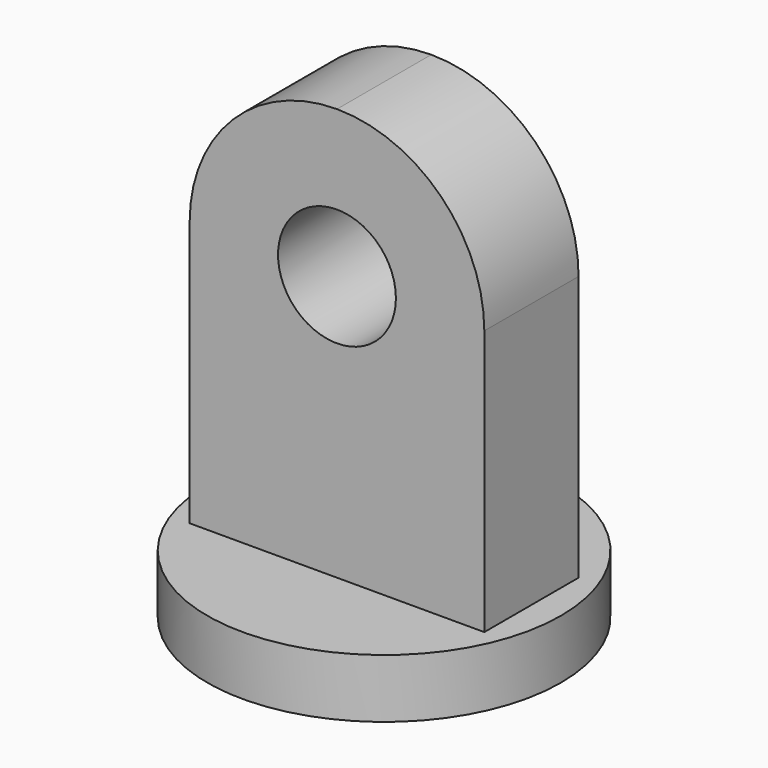
from build123d import *

# Parameters (mm, degrees)
F0_R     = 3
F1_DEPTH = 1
F2_W     = 5
F2_H     = 2
F3_DEPTH = 7
F4_R     = 2.49999
F5_R     = 1
F6_DEPTH = 4


# Not quite as in the source:
# - a fillet or chamfer is up to 0.001 mm smaller than in the source, because OpenCascade refuses the exact size


with BuildPart() as f1:
    # F0 (on Top) → F1 (new body)
    with BuildSketch(Plane.XY):
        Circle(F0_R)
    extrude(amount=F1_DEPTH)

    # F2 (on face) → F3 (join)
    with BuildSketch(Plane.XY.offset(1)):
        Rectangle(F2_W, F2_H)
    extrude(amount=F3_DEPTH)

    # F4 (radius 2.5 in the source; OpenCascade refuses exactly that, so slightly less here)
    f4_edges = [f1.edges().sort_by_distance(p)[0] for p in [
        (-2.5, 0, 8),
        (2.5, 0, 8),
    ]]
    fillet(f4_edges, radius=F4_R)

    # F5 (on face) → F6 (cut)
    with BuildSketch(Plane.XZ.offset(1)):
        with Locations((0, 5.5)):
            Circle(F5_R)
    extrude(amount=-F6_DEPTH, mode=Mode.SUBTRACT)


solid = f1.part
